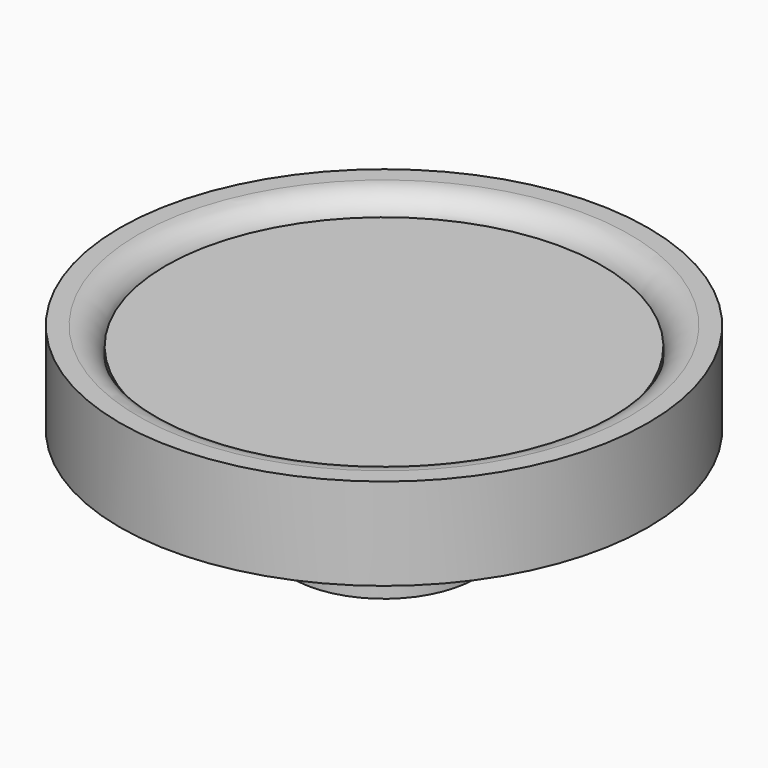
from build123d import *

# Parameters (mm, degrees)
F0_R     = 11.5
F0_R_2   = 9.5
F1_DEPTH = 4
F2_DEPTH = 3.2
F3_R     = 1.2071067812
F4_R     = 4
F5_DEPTH = 4.4


with BuildPart() as f1:
    # F0 (on Top) → F1 (new body)
    with BuildSketch(Plane.XY):
        Circle(F0_R)
        Circle(F0_R_2, mode=Mode.SUBTRACT)
    extrude(amount=F1_DEPTH)

    # F3
    f3_edges = [f1.edges().sort_by_distance(p)[0] for p in [
        (-9.5, 0, 4),
    ]]
    fillet(f3_edges, radius=F3_R)



with BuildPart() as f2:
    # F0 (on Top) → F2 (new body)
    with BuildSketch(Plane.XY):
        Circle(F0_R_2)
    extrude(amount=F2_DEPTH)


with BuildPart() as f1_1:
    add(f1.part)

    add(f2.part)  # F5 merges F2
    # F4 (on Top) → F5 (join)
    with BuildSketch(Plane.XY):
        Circle(F4_R)
    extrude(amount=-F5_DEPTH)


solid = f1_1.part
